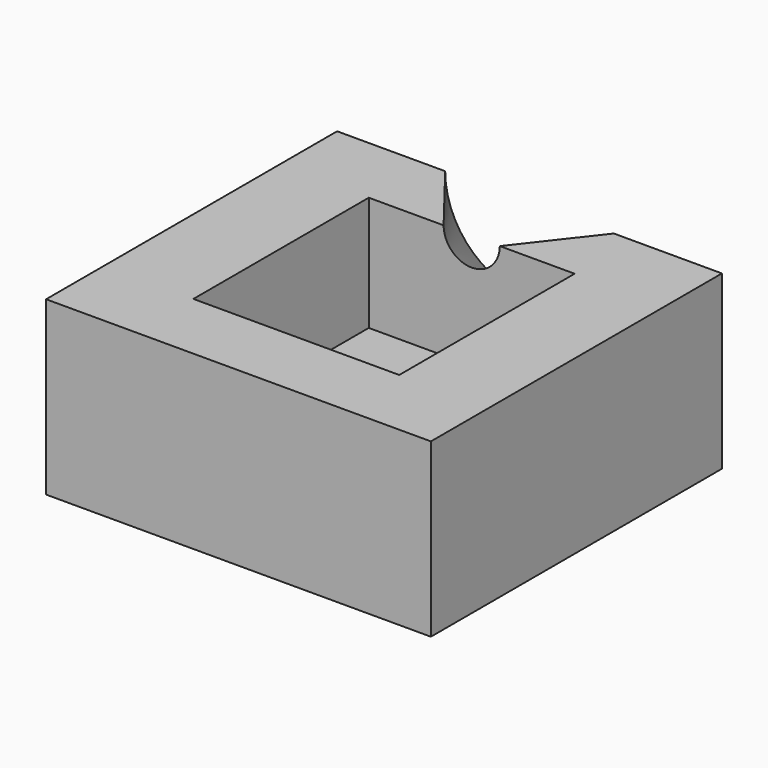
from build123d import *

# Parameters (mm, degrees)
F0_W     = 85.2533727884
F0_H     = 80.5925950408
F1_DEPTH = 38.1
F2_W     = 45.603595674
F2_H     = 48.5711470246
F3_DEPTH = 25.4


with BuildPart() as f1:
    # F0 (on Top) → F1 (new body)
    with BuildSketch(Plane.XY):
        Rectangle(F0_W, F0_H)
    extrude(amount=F1_DEPTH)

    # F2 (on face) → F3 (cut)
    with BuildSketch(Plane.XY.offset(38.1)):
        Rectangle(F2_W, F2_H)
    extrude(amount=-F3_DEPTH, mode=Mode.SUBTRACT)

    # F4 (on face) → F6 section 0
    with BuildSketch(Plane(origin=(0, 40.2962975204, 0), x_dir=(-1, 0, 0), z_dir=(0, 1, 0))):
        with BuildLine():
            Line((18.6819845074, 38.1), (-18.6819845074, 38.1))
            ThreePointArc((-18.6819845074, 38.1), (0, 19.4180154926), (18.6819845074, 38.1))
        make_face()
    # F5 (on face) → F6 section 1
    with BuildSketch(Plane.XZ.offset(-24.2855735123)):
        with BuildLine():
            Line((6.2244155373, 38.1), (-6.2244155373, 38.1))
            ThreePointArc((-6.2244155373, 38.1), (0, 31.8755844627), (6.2244155373, 38.1))
        make_face()
    loft(mode=Mode.SUBTRACT)


solid = f1.part
